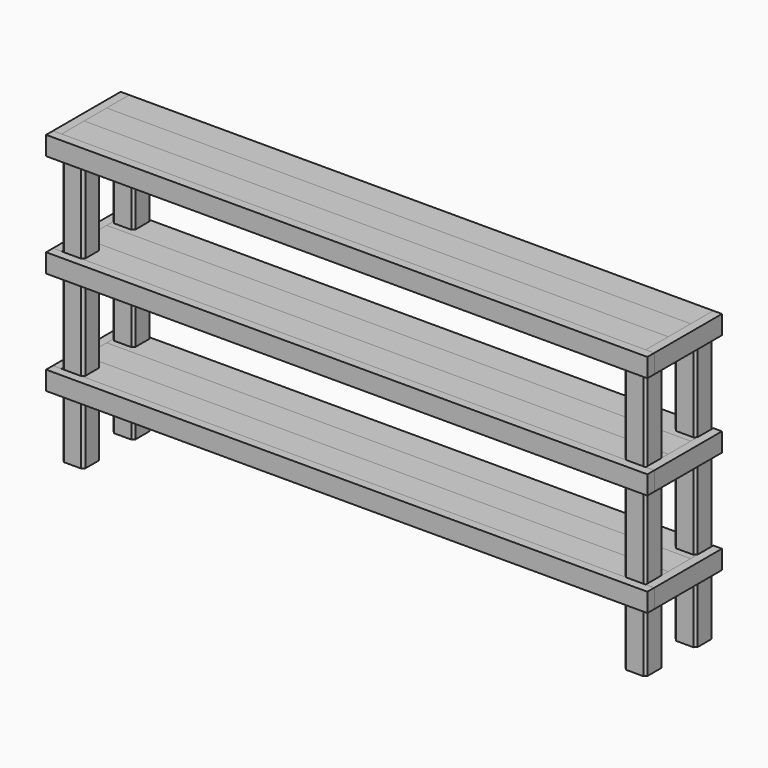
from build123d import *

# Parameters (mm, degrees)
F0_W       = 88.9
F0_H       = 88.9
F1_DEPTH   = 1168.4
F2_W       = 25.4
F2_H       = 38.1
F2_W_2     = 88.9
F3_DEPTH   = 2368.55
F2_W_3     = 114.3
F4_DEPTH   = 2368.55
F5_W       = 63.5
F5_H       = 63.5
F6_DEPTH   = 1168.401
F8_W       = 34.925
F8_H       = 76.2
F9_DEPTH   = 342.9
F10_W      = 2438.4
F10_H      = 76.2
F11_DEPTH  = 34.925
F12_SIZE   = 9.525
F12_2_SIZE = 9.525
F12_3_SIZE = 9.525
F12_4_SIZE = 9.525


with BuildPart() as f1:
    # F0 (on Top) → F1 (new body)
    with BuildSketch(Plane.XY):
        with Locations((44.45, 44.45)):
            Rectangle(F0_W, F0_H)
    extrude(amount=F1_DEPTH)


with BuildPart() as f1b:
    # F0 (on Top) → F1, piece 2 (new body)
    with BuildSketch(Plane.XY):
        with Locations((2324.1, 44.45)):
            Rectangle(F0_W, F0_H)
    extrude(amount=F1_DEPTH)


with BuildPart() as f1c:
    # F0 (on Top) → F1, piece 3 (new body)
    with BuildSketch(Plane.XY):
        with Locations((44.45, 298.45)):
            Rectangle(F0_W, F0_H)
    extrude(amount=F1_DEPTH)


with BuildPart() as f1d:
    # F0 (on Top) → F1, piece 4 (new body)
    with BuildSketch(Plane.XY):
        with Locations((2324.1, 298.45)):
            Rectangle(F0_W, F0_H)
    extrude(amount=F1_DEPTH)


with BuildPart() as f3:
    # F2 (on face) → F3 (new body, through all)
    with BuildSketch(Plane(origin=(0, 0, 0), x_dir=(0, -1, 0), z_dir=(-1, 0, 0))):
        with Locations((-241.3, 1149.35)):
            Rectangle(F2_W, F2_H)
        with Locations((-298.45, 1149.35)):
            Rectangle(F2_W_2, F2_H)
    extrude(amount=-F3_DEPTH)


with BuildPart() as f3b:
    # F2 (on face) → F3, piece 2 (new body, through all)
    with BuildSketch(Plane(origin=(0, 0, 0), x_dir=(0, -1, 0), z_dir=(-1, 0, 0))):
        with Locations((-57.15, 1149.35)):
            Rectangle(F2_W_3, F2_H)
    extrude(amount=-F3_DEPTH)


with BuildPart() as f3c:
    # F2 (on face) → F3, piece 3 (new body, through all)
    with BuildSketch(Plane(origin=(0, 0, 0), x_dir=(0, -1, 0), z_dir=(-1, 0, 0))):
        with Locations((-298.45, 730.25)):
            Rectangle(F2_W_2, F2_H)
        with Locations((-241.3, 730.25)):
            Rectangle(F2_W, F2_H)
    extrude(amount=-F3_DEPTH)


with BuildPart() as f3d:
    # F2 (on face) → F3, piece 4 (new body, through all)
    with BuildSketch(Plane(origin=(0, 0, 0), x_dir=(0, -1, 0), z_dir=(-1, 0, 0))):
        with Locations((-298.45, 311.15)):
            Rectangle(F2_W_2, F2_H)
        with Locations((-241.3, 311.15)):
            Rectangle(F2_W, F2_H)
    extrude(amount=-F3_DEPTH)


with BuildPart() as f3e:
    # F2 (on face) → F3, piece 5 (new body, through all)
    with BuildSketch(Plane(origin=(0, 0, 0), x_dir=(0, -1, 0), z_dir=(-1, 0, 0))):
        with Locations((-57.15, 311.15)):
            Rectangle(F2_W_3, F2_H)
    extrude(amount=-F3_DEPTH)


with BuildPart() as f3f:
    # F2 (on face) → F3, piece 6 (new body, through all)
    with BuildSketch(Plane(origin=(0, 0, 0), x_dir=(0, -1, 0), z_dir=(-1, 0, 0))):
        with Locations((-57.15, 730.25)):
            Rectangle(F2_W_3, F2_H)
    extrude(amount=-F3_DEPTH)


with BuildPart() as f4:
    # F2 (on face) → F4 (new body, through all)
    with BuildSketch(Plane(origin=(0, 0, 0), x_dir=(0, -1, 0), z_dir=(-1, 0, 0))):
        with Locations((-171.45, 1149.35)):
            Rectangle(F2_W_3, F2_H)
    extrude(amount=-F4_DEPTH)


with BuildPart() as f4b:
    # F2 (on face) → F4, piece 2 (new body, through all)
    with BuildSketch(Plane(origin=(0, 0, 0), x_dir=(0, -1, 0), z_dir=(-1, 0, 0))):
        with Locations((-171.45, 730.25)):
            Rectangle(F2_W_3, F2_H)
    extrude(amount=-F4_DEPTH)


with BuildPart() as f4c:
    # F2 (on face) → F4, piece 3 (new body, through all)
    with BuildSketch(Plane(origin=(0, 0, 0), x_dir=(0, -1, 0), z_dir=(-1, 0, 0))):
        with Locations((-171.45, 311.15)):
            Rectangle(F2_W_3, F2_H)
    extrude(amount=-F4_DEPTH)


with BuildPart() as f6_tool:
    # F5 (on face) → F6 (new body, through all)
    with BuildSketch(Plane.XY.offset(1168.4)):
        with Locations((31.75, 31.75)):
            Rectangle(F5_W, F5_H)
        with Locations((2336.8, 31.75)):
            Rectangle(F5_W, F5_H)
        with Locations((2336.8, 311.15)):
            Rectangle(F5_W, F5_H)
        with Locations((31.75, 311.15)):
            Rectangle(F5_W, F5_H)
    extrude(amount=-F6_DEPTH)


with BuildPart() as f3c_1:
    add(f3c.part)

    # F6: cut by f6_tool
    add(f6_tool.part, mode=Mode.SUBTRACT)


with BuildPart() as f3d_1:
    add(f3d.part)

    # F6: cut by f6_tool
    add(f6_tool.part, mode=Mode.SUBTRACT)


with BuildPart() as f3e_1:
    add(f3e.part)

    # F6: cut by f6_tool
    add(f6_tool.part, mode=Mode.SUBTRACT)


with BuildPart() as f3f_1:
    add(f3f.part)

    # F6: cut by f6_tool
    add(f6_tool.part, mode=Mode.SUBTRACT)


with BuildPart() as f1c_1:
    add(f1c.part)

    # F7: cut F3c, F3f, F3d, F3e, F3, F3b
    add(f3c_1.part, mode=Mode.SUBTRACT)
    add(f3f_1.part, mode=Mode.SUBTRACT)
    add(f3d_1.part, mode=Mode.SUBTRACT)
    add(f3e_1.part, mode=Mode.SUBTRACT)
    add(f3.part, mode=Mode.SUBTRACT)
    add(f3b.part, mode=Mode.SUBTRACT)

    # F12#3
    f12_3_edges = [f1c_1.edges().sort_by_distance(p)[0] for p in [
        (88.9, 342.9, 939.8),
        (88.9, 342.9, 520.7),
        (88.9, 342.9, 146.05),
        (88.9, 254, 146.05),
        (88.9, 254, 520.7),
        (88.9, 254, 939.8),
        (0, 254, 939.8),
        (0, 254, 520.7),
        (0, 254, 146.05),
        (0, 342.9, 565.15),
    ]]
    chamfer(f12_3_edges, length=F12_3_SIZE)


with BuildPart() as f1_1:
    add(f1.part)

    # F7: cut F3c, F3f, F3d, F3e, F3, F3b
    add(f3c_1.part, mode=Mode.SUBTRACT)
    add(f3f_1.part, mode=Mode.SUBTRACT)
    add(f3d_1.part, mode=Mode.SUBTRACT)
    add(f3e_1.part, mode=Mode.SUBTRACT)
    add(f3.part, mode=Mode.SUBTRACT)
    add(f3b.part, mode=Mode.SUBTRACT)

    # F12
    f12_edges = [f1_1.edges().sort_by_distance(p)[0] for p in [
        (0, 0, 565.15),
        (88.9, 0, 939.8),
        (88.9, 0, 520.7),
        (88.9, 0, 146.05),
        (88.9, 88.9, 146.05),
        (0, 88.9, 939.8),
        (0, 88.9, 520.7),
        (0, 88.9, 146.05),
        (88.9, 88.9, 939.8),
        (88.9, 88.9, 520.7),
    ]]
    chamfer(f12_edges, length=F12_SIZE)


with BuildPart() as f1d_1:
    add(f1d.part)

    # F7: cut F3c, F3f, F3d, F3e, F3, F3b
    add(f3c_1.part, mode=Mode.SUBTRACT)
    add(f3f_1.part, mode=Mode.SUBTRACT)
    add(f3d_1.part, mode=Mode.SUBTRACT)
    add(f3e_1.part, mode=Mode.SUBTRACT)
    add(f3.part, mode=Mode.SUBTRACT)
    add(f3b.part, mode=Mode.SUBTRACT)

    # F12#4
    f12_4_edges = [f1d_1.edges().sort_by_distance(p)[0] for p in [
        (2279.65, 254, 146.05),
        (2279.65, 254, 520.7),
        (2279.65, 254, 939.8),
        (2279.65, 342.9, 939.8),
        (2279.65, 342.9, 520.7),
        (2279.65, 342.9, 146.05),
        (2368.55, 342.9, 565.15),
        (2368.55, 254, 146.05),
        (2368.55, 254, 939.8),
        (2368.55, 254, 520.7),
    ]]
    chamfer(f12_4_edges, length=F12_4_SIZE)


with BuildPart() as f1b_1:
    add(f1b.part)

    # F7: cut F3c, F3f, F3d, F3e, F3, F3b
    add(f3c_1.part, mode=Mode.SUBTRACT)
    add(f3f_1.part, mode=Mode.SUBTRACT)
    add(f3d_1.part, mode=Mode.SUBTRACT)
    add(f3e_1.part, mode=Mode.SUBTRACT)
    add(f3.part, mode=Mode.SUBTRACT)
    add(f3b.part, mode=Mode.SUBTRACT)

    # F12#2
    f12_2_edges = [f1b_1.edges().sort_by_distance(p)[0] for p in [
        (2368.55, 88.9, 146.05),
        (2279.65, 88.9, 146.05),
        (2368.55, 88.9, 520.7),
        (2279.65, 88.9, 520.7),
        (2368.55, 88.9, 939.8),
        (2279.65, 88.9, 939.8),
        (2279.65, 0, 939.8),
        (2279.65, 0, 520.7),
        (2368.55, 0, 565.15),
        (2279.65, 0, 146.05),
    ]]
    chamfer(f12_2_edges, length=F12_2_SIZE)


with BuildPart() as f9:
    # F8 (on face) → F9 (new body, through all)
    with BuildSketch(Plane(origin=(0, 342.9, 0), x_dir=(-1, 0, 0), z_dir=(0, 1, 0))):
        with Locations((-2386.0125, 1130.3)):
            Rectangle(F8_W, F8_H)
    extrude(amount=-F9_DEPTH)


with BuildPart() as f9b:
    # F8 (on face) → F9, piece 2 (new body, through all)
    with BuildSketch(Plane(origin=(0, 342.9, 0), x_dir=(-1, 0, 0), z_dir=(0, 1, 0))):
        with Locations((-2386.0125, 711.2)):
            Rectangle(F8_W, F8_H)
    extrude(amount=-F9_DEPTH)


with BuildPart() as f9c:
    # F8 (on face) → F9, piece 3 (new body, through all)
    with BuildSketch(Plane(origin=(0, 342.9, 0), x_dir=(-1, 0, 0), z_dir=(0, 1, 0))):
        with Locations((-2386.0125, 292.1)):
            Rectangle(F8_W, F8_H)
    extrude(amount=-F9_DEPTH)


with BuildPart() as f9d:
    # F8 (on face) → F9, piece 4 (new body, through all)
    with BuildSketch(Plane(origin=(0, 342.9, 0), x_dir=(-1, 0, 0), z_dir=(0, 1, 0))):
        with Locations((17.4625, 1130.3)):
            Rectangle(F8_W, F8_H)
    extrude(amount=-F9_DEPTH)


with BuildPart() as f9e:
    # F8 (on face) → F9, piece 5 (new body, through all)
    with BuildSketch(Plane(origin=(0, 342.9, 0), x_dir=(-1, 0, 0), z_dir=(0, 1, 0))):
        with Locations((17.4625, 711.2)):
            Rectangle(F8_W, F8_H)
    extrude(amount=-F9_DEPTH)


with BuildPart() as f9f:
    # F8 (on face) → F9, piece 6 (new body, through all)
    with BuildSketch(Plane(origin=(0, 342.9, 0), x_dir=(-1, 0, 0), z_dir=(0, 1, 0))):
        with Locations((17.4625, 292.1)):
            Rectangle(F8_W, F8_H)
    extrude(amount=-F9_DEPTH)


with BuildPart() as f11:
    # F10 (on face) → F11 (new body)
    with BuildSketch(Plane.XZ):
        with Locations((1184.275, 292.1)):
            Rectangle(F10_W, F10_H)
    extrude(amount=F11_DEPTH)


with BuildPart() as f11b:
    # F10 (on face) → F11, piece 2 (new body)
    with BuildSketch(Plane.XZ):
        with Locations((1184.275, 711.2)):
            Rectangle(F10_W, F10_H)
    extrude(amount=F11_DEPTH)


with BuildPart() as f11c:
    # F10 (on face) → F11, piece 3 (new body)
    with BuildSketch(Plane.XZ):
        with Locations((1184.275, 1130.3)):
            Rectangle(F10_W, F10_H)
    extrude(amount=F11_DEPTH)


solid = Compound([f3.part, f3b.part, f4.part, f4b.part, f4c.part, f3c_1.part, f3d_1.part, f3e_1.part, f3f_1.part, f1c_1.part, f1_1.part, f1d_1.part, f1b_1.part, f9.part, f9b.part, f9c.part, f9d.part, f9e.part, f9f.part, f11.part, f11b.part, f11c.part])
